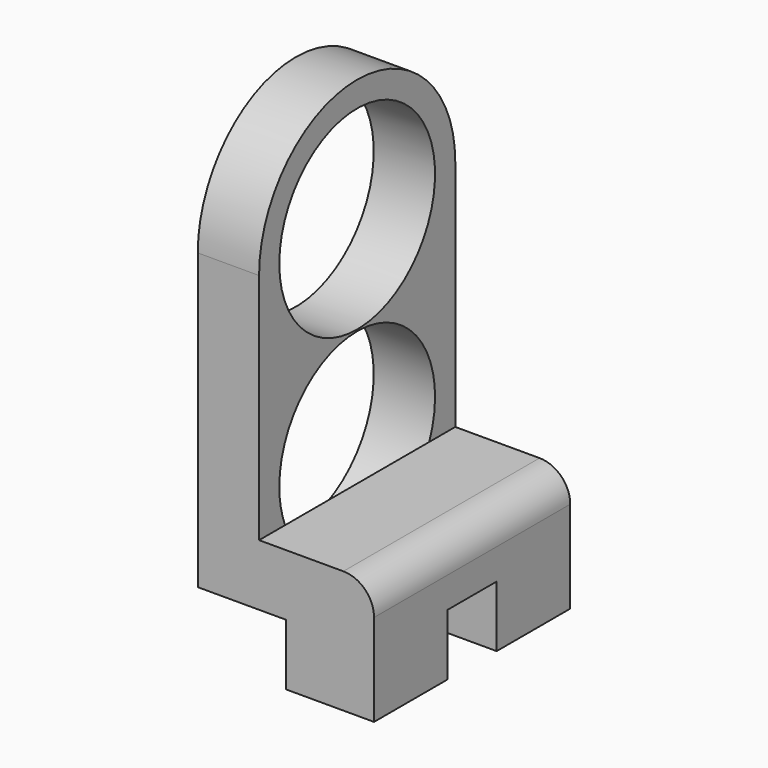
from build123d import *

# Parameters (mm, degrees)
F1_DEPTH  = 2
F2_W      = 8
F2_H      = 2
F3_DEPTH  = 3.75
F4_W      = 2.875
F4_H      = 8
F5_DEPTH  = 2
F6_W      = 2
F6_H      = 2
F7_DEPTH  = 25
F8_R      = 3.175
F9_DEPTH  = 2
F10_R     = 3.175
F11_DEPTH = 2
F12_R     = 1


with BuildPart() as f1:
    # F0 (on Right) → F1 (new body)
    with BuildSketch(Plane.YZ):
        with BuildLine():
            Line((-4, 9.6), (4, 9.6))
            ThreePointArc((4, 9.6), (0, 13.6), (-4, 9.6))
        make_face()
        with BuildLine():
            ThreePointArc((-4, 9.6), (0, 5.6), (4, 9.6))
            Line((4, 9.6), (-4, 9.6))
        make_face()
        with BuildLine():
            Line((4, 0), (4, 9.6))
            ThreePointArc((4, 9.6), (0, 5.6), (-4, 9.6))
            Line((-4, 9.6), (-4, 0))
            Line((-4, 0), (4, 0))
        make_face()
    extrude(amount=F1_DEPTH)

    # F2 (on face) → F3 (join)
    with BuildSketch(Plane.YZ.offset(2)):
        with Locations((0, 1)):
            Rectangle(F2_W, F2_H)
    extrude(amount=F3_DEPTH)

    # F4 (on face) → F5 (join)
    with BuildSketch(Plane(origin=(0, 0, 0), x_dir=(1, 0, 0), z_dir=(0, 0, -1))):
        with Locations((4.3125, 0)):
            Rectangle(F4_W, F4_H)
    extrude(amount=F5_DEPTH)

    # F6 (on face) → F7 (cut)
    with BuildSketch(Plane.YZ.offset(5.75)):
        with Locations((0, -1)):
            Rectangle(F6_W, F6_H)
    extrude(amount=-F7_DEPTH, mode=Mode.SUBTRACT)

    # F8 (on face) → F9 (cut)
    with BuildSketch(Plane(origin=(0, 0, 0), x_dir=(0, -1, 0), z_dir=(-1, 0, 0))):
        with Locations((0, 9.6)):
            Circle(F8_R)
    extrude(amount=-F9_DEPTH, mode=Mode.SUBTRACT)

    # F10 (on face) → F11 (cut)
    with BuildSketch(Plane(origin=(0, 0, 0), x_dir=(0, -1, 0), z_dir=(-1, 0, 0))):
        with Locations((0, 3.2)):
            Circle(F10_R)
    extrude(amount=-F11_DEPTH, mode=Mode.SUBTRACT)

    # F12
    f12_edges = [f1.edges().sort_by_distance(p)[0] for p in [
        (5.75, 0, 2),
    ]]
    fillet(f12_edges, radius=F12_R)


solid = f1.part
